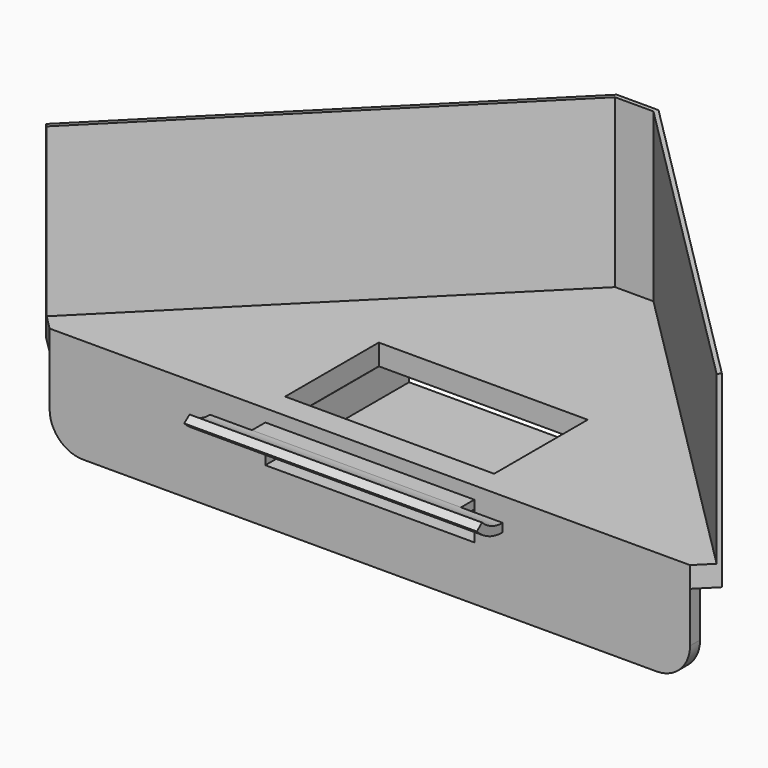
from build123d import *

# Parameters (mm, degrees)
F1_DEPTH         = 3.175
F3_DEPTH         = 25.4
F4_W             = 97.3040463274
F4_H             = 1.905
F5_DEPTH         = 12.7
F6_W             = 40.64
F6_H             = 25.4
F7_DEPTH         = 11.43
F8_W             = 31.75
F8_H             = 17.78
F9_DEPTH         = 3.175
F10_W            = 31.75
F10_H            = 4.445
F11_DEPTH        = 27.305
F12_W            = 31.75
F12_H            = 1.27
F13_DEPTH        = 2.54
F15_DEPTH        = 31.75
F15_COPIES_COUNT = 3
F15_COPIES_PITCH = 0.5207
F17_DEPTH        = 38.1
F18_DEPTH        = 6.35
F19_R            = 5.08


# Not quite as in the source:
# - a pattern or mirror of a feature is missing from the dataset's text; its kind, count and spacing are read off the source's solid


with BuildPart() as f1:
    # F0 (on Top) → F1 (new body)
    with BuildSketch(Plane.XY):
        Polygon((3.175, 48.1711), (-3.175, 48.1711), (-51.3461, 0), (-48.6520231637, -2.6940768363), (48.6520231637, -2.6940768363), (51.3461, 0), align=None)
    extrude(amount=F1_DEPTH)

    # F2 (on face) → F3 (join)
    with BuildSketch(Plane.XY.offset(3.175)):
        Polygon((-3.175, 48.1711), (-51.3461, 0), (-50.8970871939, -0.4490128061), (-2.916877582, 47.5311968059), (2.916871896, 47.5312024919), (50.8970871939, -0.4490128061), (51.3461, 0), (3.175, 48.1711), align=None)
    extrude(amount=F3_DEPTH)

    # F4 (on face) → F5 (join)
    with BuildSketch(Plane(origin=(0, 0, 0), x_dir=(1, 0, 0), z_dir=(0, 0, -1))):
        with Locations((0, 1.7415768363)):
            Rectangle(F4_W, F4_H)
    extrude(amount=F5_DEPTH)

    # F6 (on face) → F7 (join)
    with BuildSketch(Plane(origin=(0, 0, 0), x_dir=(1, 0, 0), z_dir=(0, 0, -1))):
        with Locations((-0.0357092768, -11.9109231637)):
            Rectangle(F6_W, F6_H)
    extrude(amount=F7_DEPTH)

    # F8 (on face) → F9 (cut, through all)
    with BuildSketch(Plane(origin=(0, 0, 0), x_dir=(1, 0, 0), z_dir=(0, 0, -1))):
        with Locations((-0.0357092768, -10.0059231637)):
            Rectangle(F8_W, F8_H)
    extrude(amount=-F9_DEPTH, mode=Mode.SUBTRACT)

    # F10 (on face) → F11 (cut, through all)
    with BuildSketch(Plane(origin=(0, 24.6109231637, 0), x_dir=(-1, 0, 0), z_dir=(0, 1, 0))):
        with Locations((-7.74733e-05, -2.2225)):
            Rectangle(F10_W, F10_H)
    extrude(amount=-F11_DEPTH, mode=Mode.SUBTRACT)

    # F12 (on face) → F13 (join)
    with BuildSketch(Plane.XZ.offset(2.6940768363)):
        with Locations((7.74733e-05, 0.635)):
            Rectangle(F12_W, F12_H)
    extrude(amount=F13_DEPTH)

    # F14 (on face) → F15 (join, through all)
    with BuildSketch(Plane.YZ.offset(15.8750774733)):
        Polygon((-3.6032828125, -0.3642210371), (-3.0831212644, 0), (-3.6032828125, 0), align=None)
    f15 = extrude(amount=-F15_DEPTH)

    # F15_copies: F15 ×3
    with Locations(*[(0, -i * F15_COPIES_PITCH, 0) for i in range(1, F15_COPIES_COUNT)]):
        add(f15)

    # F16 (on face) → F17 (join)
    with BuildSketch(Plane.YZ.offset(15.8750774733)):
        with BuildLine():
            Line((-9.1575253509, 2.9035897025), (-10.161578661, 2.1184348754))
            ThreePointArc((-10.161578661, 2.1184348754), (-7.9158691733, 0.5520507884), (-5.2340768363, 0))
            Line((-5.2340768363, 0), (-5.2340768363, 1.27))
            ThreePointArc((-5.2340768363, 1.27), (-7.3590511634, 1.6947115498), (-9.1575253509, 2.9035897025))
        make_face()
    extrude(amount=-F17_DEPTH)

    # F16 (on face) → F18 (join)
    with BuildSketch(Plane.YZ.offset(15.8750774733)):
        with BuildLine():
            Line((-9.1575253509, 2.9035897025), (-10.161578661, 2.1184348754))
            ThreePointArc((-10.161578661, 2.1184348754), (-7.9158691733, 0.5520507884), (-5.2340768363, 0))
            Line((-5.2340768363, 0), (-5.2340768363, 1.27))
            ThreePointArc((-5.2340768363, 1.27), (-7.3590511634, 1.6947115498), (-9.1575253509, 2.9035897025))
        make_face()
    extrude(amount=F18_DEPTH)

    # F19
    f19_edges = [f1.edges().sort_by_distance(p)[0] for p in [
        (-48.652023, -1.741577, -12.7),
        (48.652023, -1.741577, -12.7),
    ]]
    fillet(f19_edges, radius=F19_R)


solid = f1.part
